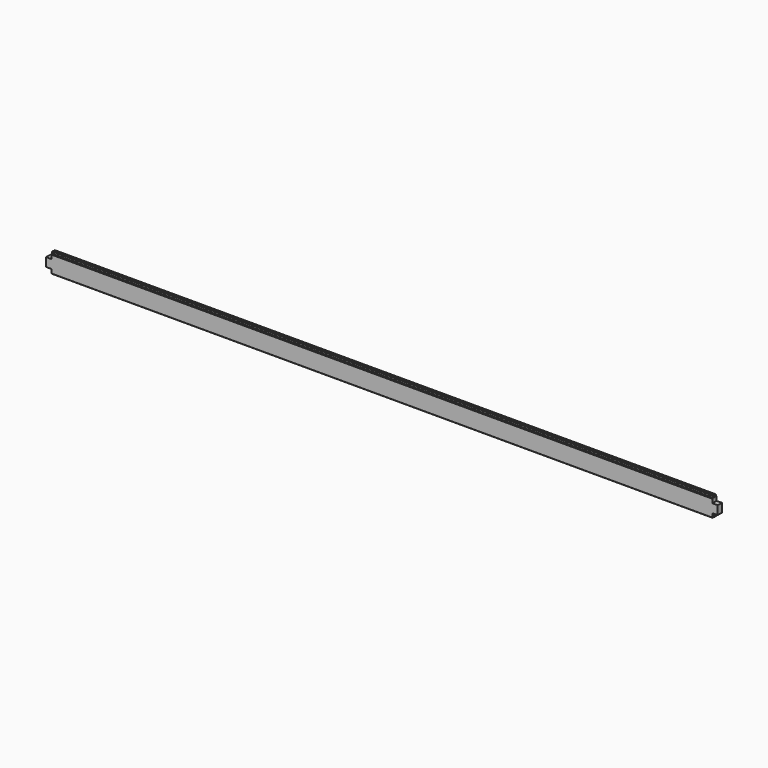
from build123d import *

# Parameters (mm, degrees)
F1_W     = 40
F1_H     = 33
F3_DEPTH = 2550
F2_W     = 80
F2_H     = 100
F4_DEPTH = 25


with BuildPart() as f3:
    # F1 (on Right) → F3 (new body, symmetric)
    with BuildSketch(Plane.YZ):
        Polygon((20, 33), (20, 63), (17, 66), (12, 66), (12, 80), (4, 80), (4, 66), (-4, 66), (-4, 80), (-12, 80), (-12, 66), (-17, 66), (-20, 63), (-20, 33), align=None)
        with Locations((0, 16.5)):
            Rectangle(F1_W, F1_H)
        with Locations((0, -16.5)):
            Rectangle(F1_W, F1_H)
        Polygon((20, -63), (20, -33), (-20, -33), (-20, -63), (-17, -66), (-12, -66), (-12, -52), (-4, -52), (-4, -66), (4, -66), (4, -52), (12, -52), (12, -66), (17, -66), align=None)
    extrude(amount=F3_DEPTH, both=True)

    # F2 (on Front) → F4 (cut, symmetric)
    with BuildSketch(Plane.XZ):
        with Locations((-2550, 83)):
            Rectangle(F2_W, F2_H)
        with Locations((-2550, -83)):
            Rectangle(F2_W, F2_H)
        with Locations((2550, 83)):
            Rectangle(F2_W, F2_H)
        with Locations((2550, -83)):
            Rectangle(F2_W, F2_H)
    extrude(amount=F4_DEPTH, both=True, mode=Mode.SUBTRACT)


solid = f3.part
